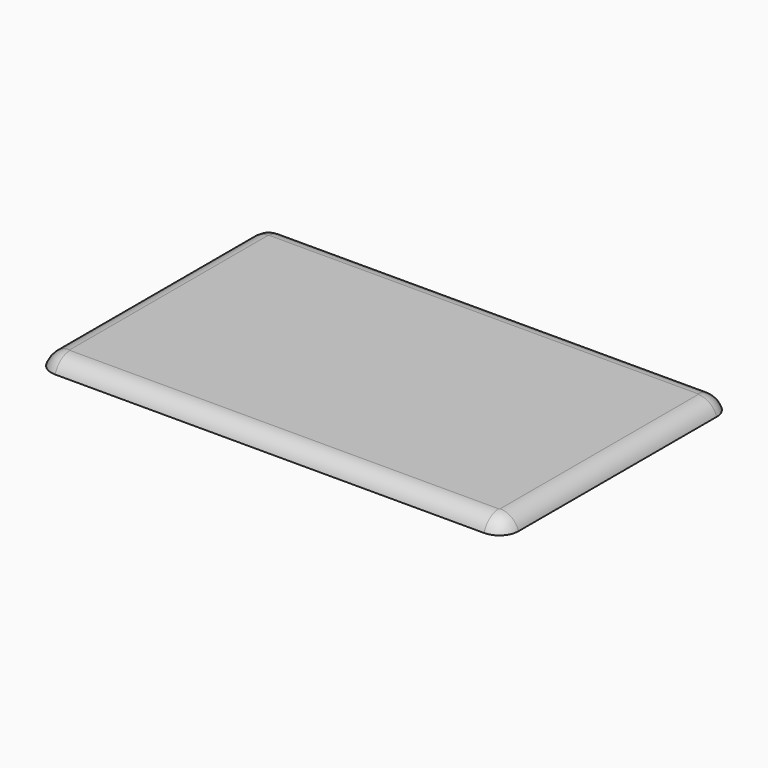
from build123d import *

# Parameters (mm, degrees)
F0_W         = 124.0848004818
F0_H         = 75.9339258075
F1_DEPTH     = 3.6583524197
F2_R         = 5.08
F3_T1_DEPTH  = 113.9248004818
F3_T3_DEPTH  = 65.7739258075
F3_T6_ANGLE  = 90
F3_T8_ANGLE  = 90
F3_T10_ANGLE = 90
F3_T12_ANGLE = 90


# Not quite as in the source:
# - a fillet or chamfer that OpenCascade refuses, or shapes differently, is made with other operations: its cross-section is extruded or revolved along the edge and cut away or added


with BuildPart() as f1:
    # F0 (on Top) → F1 (new body)
    with BuildSketch(Plane.XY):
        with Locations((-32.2462767363, 8.972465992)):
            Rectangle(F0_W, F0_H)
    extrude(amount=-F1_DEPTH)

    # F2
    f2_edges = [f1.edges().sort_by_distance(p)[0] for p in [
        (29.796124, 46.939429, -1.829176),
        (29.796124, -28.994497, -1.829176),
        (-94.288677, 46.939429, -1.829176),
        (-94.288677, -28.994497, -1.829176),
    ]]
    fillet(f2_edges, radius=F2_R)

    # F3: fillet of radius 5.08 on 1 edges, made by hand

    # F3_s2 → F3_t1 (cut)
    with BuildSketch(Plane.YZ.offset(-89.2086769772)):
        with BuildLine():
            ThreePointArc((42.0624095029, 0), (45.110722995, -1.016235138), (46.9394288957, -3.6583524197))
            Line((46.9394288957, -3.6583524197), (46.9394288957, 0))
            Line((46.9394288957, 0), (42.0624095029, 0))
        make_face()
        with BuildLine():
            ThreePointArc((-24.117477519, 0), (-27.1657910111, -1.016235138), (-28.9944969118, -3.6583524197))
            Line((-28.9944969118, -3.6583524197), (-28.9944969118, 0))
            Line((-28.9944969118, 0), (-24.117477519, 0))
        make_face()
    extrude(amount=F3_T1_DEPTH, mode=Mode.SUBTRACT)

    # F3_s4 → F3_t3 (cut)
    with BuildSketch(Plane.XZ.offset(-41.8594288957)):
        with BuildLine():
            ThreePointArc((-89.4116575844, 0), (-92.4599710765, -1.016235138), (-94.2886769772, -3.6583524197))
            Line((-94.2886769772, -3.6583524197), (-94.2886769772, 0))
            Line((-94.2886769772, 0), (-89.4116575844, 0))
        make_face()
        with BuildLine():
            ThreePointArc((29.7961235046, -3.6583524197), (27.967417604, -1.016235138), (24.9191041119, 0))
            Line((24.9191041119, 0), (29.7961235046, 0))
            Line((29.7961235046, 0), (29.7961235046, -3.6583524197))
        make_face()
    extrude(amount=F3_T3_DEPTH, mode=Mode.SUBTRACT)

    # F3_s5 → F3_t6 (revolve, cut)
    with BuildSketch(Plane.YZ.offset(-89.2086769772)):
        with BuildLine():
            ThreePointArc((42.0624095029, 0), (45.110722995, -1.016235138), (46.9394288957, -3.6583524197))
            Line((46.9394288957, -3.6583524197), (46.9394288957, 0))
            Line((46.9394288957, 0), (42.0624095029, 0))
        make_face()
    revolve(axis=Axis((-89.2086769772, 41.8594288957, 0), (0, 0, 1)), revolution_arc=F3_T6_ANGLE, mode=Mode.SUBTRACT)

    # F3_s7 → F3_t8 (revolve, cut)
    with BuildSketch(Plane.XZ.offset(23.9144969118)):
        with BuildLine():
            ThreePointArc((-89.4116575844, 0), (-92.4599710765, -1.016235138), (-94.2886769772, -3.6583524197))
            Line((-94.2886769772, -3.6583524197), (-94.2886769772, 0))
            Line((-94.2886769772, 0), (-89.4116575844, 0))
        make_face()
    revolve(axis=Axis((-89.2086769772, -23.9144969118, 0), (0, 0, 1)), revolution_arc=F3_T8_ANGLE, mode=Mode.SUBTRACT)

    # F3_s9 → F3_t10 (revolve, cut)
    with BuildSketch(Plane.XZ.offset(23.9144969118)):
        with BuildLine():
            ThreePointArc((24.9191041119, 0), (27.967417604, -1.016235138), (29.7961235046, -3.6583524197))
            Line((29.7961235046, -3.6583524197), (29.7961235046, 0))
            Line((29.7961235046, 0), (24.9191041119, 0))
        make_face()
    revolve(axis=Axis((24.7161235046, -23.9144969118, 0), (0, 0, -1)), revolution_arc=F3_T10_ANGLE, mode=Mode.SUBTRACT)

    # F3_s11 → F3_t12 (revolve, cut)
    with BuildSketch(Plane.XZ.offset(-41.8594288957)):
        with BuildLine():
            ThreePointArc((24.9191041119, 0), (27.967417604, -1.016235138), (29.7961235046, -3.6583524197))
            Line((29.7961235046, -3.6583524197), (29.7961235046, 0))
            Line((29.7961235046, 0), (24.9191041119, 0))
        make_face()
    revolve(axis=Axis((24.7161235046, 41.8594288957, 0), (0, 0, 1)), revolution_arc=F3_T12_ANGLE, mode=Mode.SUBTRACT)


solid = f1.part
